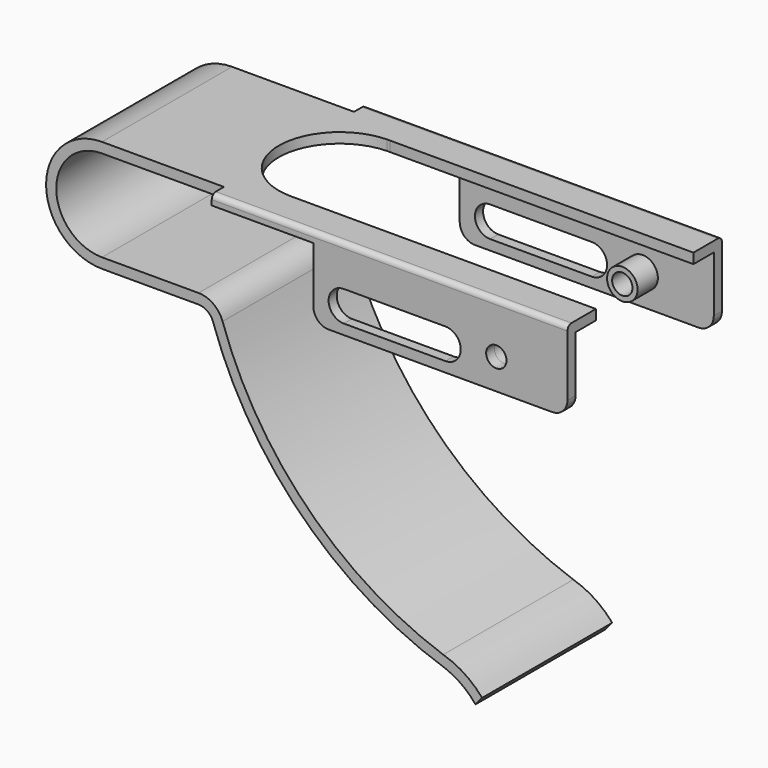
from build123d import *

# Parameters (mm, degrees)
F1_DEPTH  = 16
F2_W      = 70
F2_H      = 3
F3_DEPTH  = 2
F4_W      = 50
F4_H      = 14
F5_DEPTH  = 2
F6_R      = 1
F9_DEPTH  = 2
F11_DEPTH = 38.001
F13_D     = 4
F14_R     = 2.999996841
F14_R_2   = 2
F15_DEPTH = 5
F16_R     = 3


# Not quite as in the source:
# - a pattern or mirror of a feature is missing from the dataset's text; its kind, count and spacing are read off the source's solid


with BuildPart() as f1:
    # F0 (on Front) → F1 (new body)
    with BuildSketch(Plane.XZ):
        with BuildLine():
            ThreePointArc((0, -9), (-9, 0), (0, 9))
            Line((0, 9), (94, 9))
            Line((94, 9), (94, 11))
            Line((94, 11), (0, 11))
            ThreePointArc((0, 11), (-11, 0), (0, -11))
            Line((0, -11), (19, -11))
            ThreePointArc((19, -11), (20.7464347921, -11.5607448848), (21.84, -13.0333563221))
            ThreePointArc((21.84, -13.0333563221), (39.3752187726, -41.0308955197), (67.5680682322, -58.2503420228))
            ThreePointArc((67.5680682322, -58.2503420228), (70.8216506695, -60.0087849904), (73.5012506711, -62.5578366136))
            Line((73.5012506711, -62.5578366136), (74.808430799, -61))
            ThreePointArc((74.808430799, -61), (71.3448519203, -57.9413219983), (67.1516242057, -56))
            ThreePointArc((67.1516242057, -56), (40.3930033582, -39.2216179023), (23.7333333333, -12.3889272035))
            ThreePointArc((23.7333333333, -12.3889272035), (21.9107246536, -9.9345748081), (19, -9))
            Line((19, -9), (0, -9))
        make_face()
    extrude(amount=F1_DEPTH)

    # F2 (on face) → F3 (join)
    with BuildSketch(Plane.XY.offset(11)):
        with Locations((59, -17.5)):
            Rectangle(F2_W, F2_H)
    extrude(amount=-F3_DEPTH)

    # F4 (on face) → F5 (join)
    with BuildSketch(Plane.XZ.offset(19)):
        with Locations((69, 2)):
            Rectangle(F4_W, F4_H)
    extrude(amount=-F5_DEPTH)

    # F6
    f6_edges = [f1.edges().sort_by_distance(p)[0] for p in [
        (59, -19, 11),
    ]]
    fillet(f6_edges, radius=F6_R)

    # F7: F1 across plane


with BuildPart() as f1_1:
    add(f1.part)
    add(f1.part.mirror(Plane.XZ))

    # F8 (on face) → F9 (cut)
    with BuildSketch(Plane.XY.offset(11)):
        with BuildLine():
            Line((33.7271293001, 11.9968971647), (34.2728706999, 11.9968971647))
            ThreePointArc((34.2728706999, 11.9968971647), (34, 12), (33.7271293001, 11.9968971647))
        make_face()
        with BuildLine():
            Line((94, 11.9968971647), (34.2728706999, 11.9968971647))
            Line((34.2728706999, 11.9968971647), (33.7271293001, 11.9968971647))
            ThreePointArc((33.7271293001, 11.9968971647), (22.0007757339, -0.1364441703), (34, -12))
            Line((34, -12), (94, -12))
            Line((94, -12), (94, 11.9968971647))
        make_face()
    extrude(amount=-F9_DEPTH, mode=Mode.SUBTRACT)

    # F10 (on face) → F11 (cut, through all)
    with BuildSketch(Plane.XZ.offset(19)):
        with BuildLine():
            ThreePointArc((50, 3), (47, 0), (50, -3))
            Line((50, -3), (70, -3))
            ThreePointArc((70, -3), (73, 0), (70, 3))
            Line((70, 3), (50, 3))
        make_face()
    extrude(amount=-F11_DEPTH, mode=Mode.SUBTRACT)

    # F13 (through all)
    with Locations(Plane.XZ.offset(19)):
        with Locations((80, 1)):
            Hole(F13_D / 2)

    # F14 (on face) → F15 (join)
    with BuildSketch(Plane(origin=(0, -17, 0), x_dir=(-1, 0, 0), z_dir=(0, 1, 0))):
        with Locations((-80, 1)):
            Circle(F14_R)
        with Locations((-80, 1)):
            Circle(F14_R_2, mode=Mode.SUBTRACT)
    f15 = extrude(amount=F15_DEPTH)

    # F15_copies: F15 across plane
    add(f15.mirror(Plane.ZX))

    # F16
    f16_edges = [f1_1.edges().sort_by_distance(p)[0] for p in [
        (94, -18, -5),
        (44, -18, -5),
        (94, 18, -5),
        (44, 18, -5),
    ]]
    fillet(f16_edges, radius=F16_R)


solid = f1_1.part
